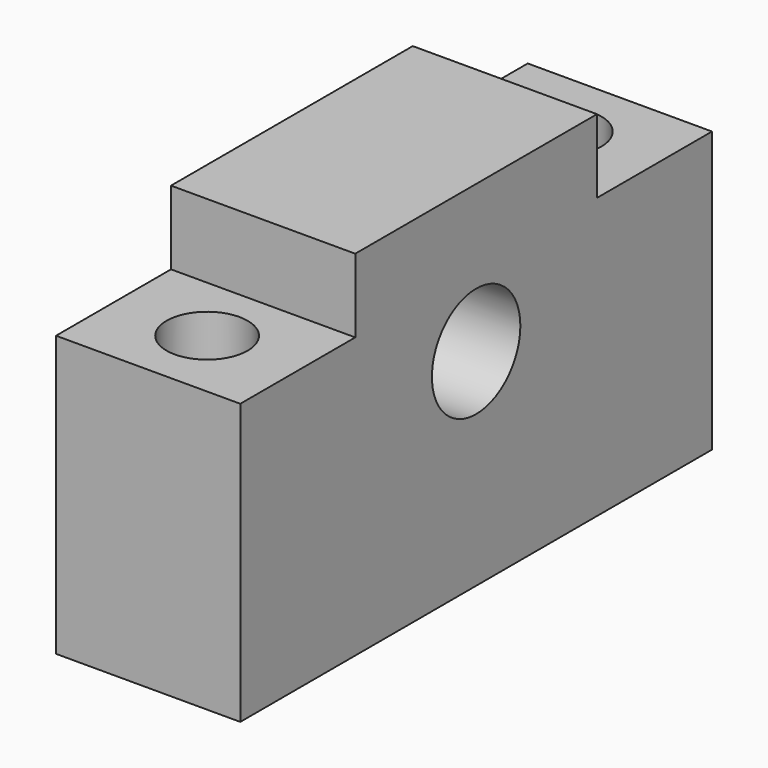
from build123d import *

# Parameters (mm, degrees)
F0_W     = 80
F0_H     = 48
F1_DEPTH = 25
F2_W     = 19.5
F2_H     = 10
F3_DEPTH = 25.001
F4_R     = 7.5
F5_DEPTH = 25.001
F6_R     = 5.5
F6_R_2   = 4
F7_DEPTH = 25
F8_DEPTH = 38.001


with BuildPart() as f1:
    # F0 (on Right) → F1 (new body)
    with BuildSketch(Plane.YZ):
        Rectangle(F0_W, F0_H)
    extrude(amount=-F1_DEPTH)

    # F2 (on face) → F3 (cut, through all)
    with BuildSketch(Plane.YZ):
        with Locations((-30.25, 19)):
            Rectangle(F2_W, F2_H)
        with Locations((30.25, 19)):
            Rectangle(F2_W, F2_H)
    extrude(amount=-F3_DEPTH, mode=Mode.SUBTRACT)

    # F4 (on face) → F5 (cut, through all)
    with BuildSketch(Plane.YZ):
        with Locations((0, 4)):
            Circle(F4_R)
    extrude(amount=-F5_DEPTH, mode=Mode.SUBTRACT)

    # F6 (on face) → F7 (cut)
    with BuildSketch(Plane.XY.offset(14)):
        with Locations((-12.5, 30)):
            Circle(F6_R)
        with Locations((-12.5, 30)):
            Circle(F6_R_2, mode=Mode.SUBTRACT)
        with Locations((-12.5, -30)):
            Circle(F6_R)
        with Locations((-12.5, -30)):
            Circle(F6_R_2, mode=Mode.SUBTRACT)
    extrude(amount=-F7_DEPTH, mode=Mode.SUBTRACT)

    # F8 (cut, through all): faces of the model
    f8_faces = [f1.faces().sort_by_distance(p)[0] for p in [
        (-12.5, 30, 14),
        (-12.5, -30, 14),
    ]]
    extrude(f8_faces, amount=-F8_DEPTH, mode=Mode.SUBTRACT)


solid = f1.part
